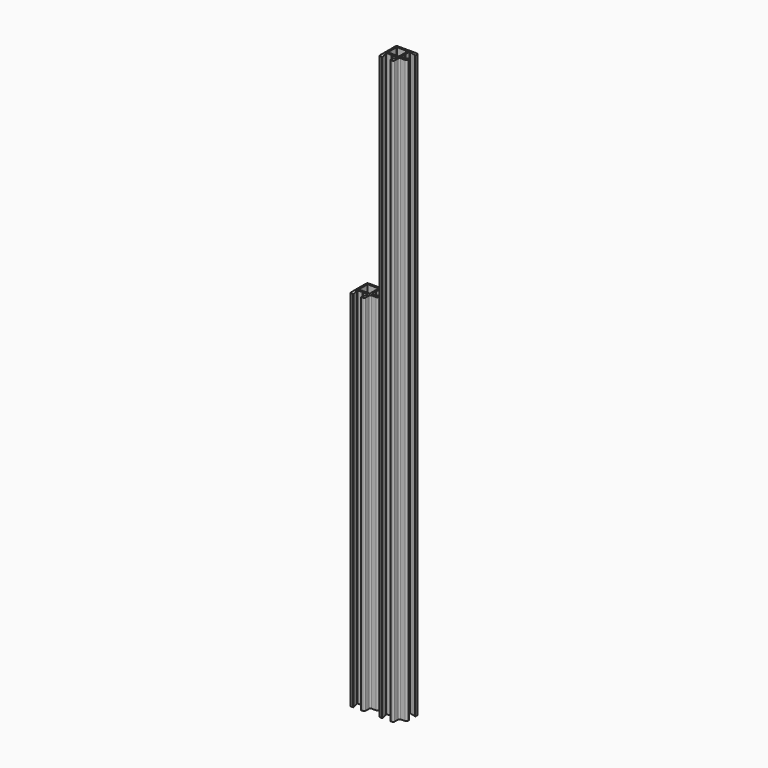
from build123d import *

# Parameters (mm, degrees)
F1_DEPTH = 1000
F2_DEPTH = 1600


# Not quite as in the source:
# - ends of sketch curves that miss each other by under 0.0002 mm in the source are joined


with BuildPart() as f1:
    # F0 (on Top) → F1 (new body)
    with BuildSketch(Plane.XY):
        with BuildLine():
            ThreePointArc((30, -1.879032), (29.5109517857, -0.8873403242), (28.4264761923, -0.6716247175))
            Line((28.4264761923, -0.6716247175), (11.258819, -5.271684))
            ThreePointArc((11.258819, -5.271684), (10.3912385359, -5.0991113133), (10, -4.305758))
            Line((10, -4.305758), (10, 9))
            ThreePointArc((10, 9), (9.9829629324, 9.1294094506), (9.9330127764, 9.2499998709))
            Line((9.9330127764, 9.2499998709), (9.644338, 9.75))
            ThreePointArc((9.644338, 9.75), (9.57735, 10), (9.6443374736, 10.2500003039))
            Line((9.6443374736, 10.2500003039), (9.933013, 10.75))
            ThreePointArc((9.933013, 10.75), (9.9829629324, 10.8705905494), (10, 11))
            Line((10, 11), (10, 24.305758))
            ThreePointArc((10, 24.305758), (10.3912385359, 25.0991113133), (11.2588189596, 25.2716838492))
            Line((11.2588189596, 25.2716838492), (28.426476, 20.671624))
            ThreePointArc((28.426476, 20.671624), (29.5109517857, 20.8873403242), (30, 21.879032))
            Line((30, 21.879032), (30, 26))
            ThreePointArc((30, 26), (28.8284271247, 28.8284271247), (26, 30))
            Line((26, 30), (-26, 30))
            ThreePointArc((-26, 30), (-28.8284271247, 28.8284271247), (-30, 26))
            Line((-30, 26), (-30, -26))
            ThreePointArc((-30, -26), (-28.8284271247, -28.8284271247), (-26, -30))
            Line((-26, -30), (-21.879032, -30))
            ThreePointArc((-21.879032, -30), (-20.8873403242, -29.5109517857), (-20.6716247175, -28.4264761923))
            Line((-20.6716247175, -28.4264761923), (-25.271684, -11.258819))
            ThreePointArc((-25.271684, -11.258819), (-25.0991113133, -10.3912385359), (-24.305758, -10))
            Line((-24.305758, -10), (-11, -10))
            ThreePointArc((-11, -10), (-10.8705905494, -9.9829629324), (-10.7500001291, -9.9330127764))
            Line((-10.7500001291, -9.9330127764), (-10.25, -9.644338))
            ThreePointArc((-10.25, -9.644338), (-10, -9.57735), (-9.7499996961, -9.6443374736))
            Line((-9.7499996961, -9.6443374736), (-9.25, -9.933013))
            ThreePointArc((-9.25, -9.933013), (-9.1294094506, -9.9829629324), (-9, -10))
            Line((-9, -10), (4.305758, -10))
            ThreePointArc((4.305758, -10), (5.0991113133, -10.3912385359), (5.2716838492, -11.2588189596))
            Line((5.2716838492, -11.2588189596), (0.671624, -28.426476))
            ThreePointArc((0.671624, -28.426476), (0.8873403242, -29.5109517857), (1.879032, -30))
            Line((1.879032, -30), (6, -30))
            ThreePointArc((6, -30), (8.8284271247, -28.8284271247), (10, -26))
            Line((10, -26), (10, -14))
            ThreePointArc((10, -14), (11.1715728753, -11.1715728753), (14, -10))
            Line((14, -10), (26, -10))
            ThreePointArc((26, -10), (28.8284271247, -8.8284271247), (30, -6))
            Line((30, -6), (30, -1.879032))
        make_face()
        with BuildLine():
            Line((5.25, 24.75), (5.25, -4.75))
            ThreePointArc((5.25, -4.75), (5.1035533906, -5.1035533906), (4.75, -5.25))
            Line((4.75, -5.25), (-24.75, -5.25))
            ThreePointArc((-24.75, -5.25), (-25.1035533906, -5.1035533906), (-25.25, -4.75))
            Line((-25.25, -4.75), (-25.25, 24.75))
            ThreePointArc((-25.25, 24.75), (-25.1035533906, 25.1035533906), (-24.75, 25.25))
            Line((-24.75, 25.25), (4.75, 25.25))
            ThreePointArc((4.75, 25.25), (5.1035533906, 25.1035533906), (5.25, 24.75))
        make_face(mode=Mode.SUBTRACT)
    extrude(amount=F1_DEPTH)


with BuildPart() as f2:
    # F0 (on Top) → F2 (new body)
    with BuildSketch(Plane.XY):
        with BuildLine():
            ThreePointArc((110, -1.879032), (109.5109517857, -0.8873403242), (108.4264761923, -0.6716247175))
            Line((108.4264761923, -0.6716247175), (91.258819, -5.271684))
            ThreePointArc((91.258819, -5.271684), (90.3912385359, -5.0991113133), (90, -4.305758))
            Line((90, -4.305758), (90, 9))
            ThreePointArc((90, 9), (89.9829629324, 9.1294094506), (89.9330127764, 9.2499998709))
            Line((89.9330127764, 9.2499998709), (89.644338, 9.75))
            ThreePointArc((89.644338, 9.75), (89.57735, 10), (89.6443374736, 10.2500003039))
            Line((89.6443374736, 10.2500003039), (89.933013, 10.75))
            ThreePointArc((89.933013, 10.75), (89.9829629324, 10.8705905494), (90, 11))
            Line((90, 11), (90, 24.305758))
            ThreePointArc((90, 24.305758), (90.3912385359, 25.0991113133), (91.2588189596, 25.2716838492))
            Line((91.2588189596, 25.2716838492), (108.426476, 20.671624))
            ThreePointArc((108.426476, 20.671624), (109.5109517857, 20.8873403242), (110, 21.879032))
            Line((110, 21.879032), (110, 26))
            ThreePointArc((110, 26), (108.8284271247, 28.8284271247), (106, 30))
            Line((106, 30), (54, 30))
            ThreePointArc((54, 30), (51.1715728753, 28.8284271247), (50, 26))
            Line((50, 26), (50, -26))
            ThreePointArc((50, -26), (51.1715728753, -28.8284271247), (54, -30))
            Line((54, -30), (58.120968, -30))
            ThreePointArc((58.120968, -30), (59.1126596758, -29.5109517857), (59.3283752825, -28.4264761923))
            Line((59.3283752825, -28.4264761923), (54.728316, -11.258819))
            ThreePointArc((54.728316, -11.258819), (54.9008886867, -10.3912385359), (55.694242, -10))
            Line((55.694242, -10), (69, -10))
            ThreePointArc((69, -10), (69.1294094506, -9.9829629324), (69.2499998709, -9.9330127764))
            Line((69.2499998709, -9.9330127764), (69.75, -9.644338))
            ThreePointArc((69.75, -9.644338), (70, -9.57735), (70.2500003039, -9.6443374736))
            Line((70.2500003039, -9.6443374736), (70.75, -9.933013))
            ThreePointArc((70.75, -9.933013), (70.8705905494, -9.9829629324), (71, -10))
            Line((71, -10), (84.305758, -10))
            ThreePointArc((84.305758, -10), (85.0991113133, -10.3912385359), (85.2716838492, -11.2588189596))
            Line((85.2716838492, -11.2588189596), (80.671624, -28.426476))
            ThreePointArc((80.671624, -28.426476), (80.8873403242, -29.5109517857), (81.879032, -30))
            Line((81.879032, -30), (86, -30))
            ThreePointArc((86, -30), (88.8284271247, -28.8284271247), (90, -26))
            Line((90, -26), (90, -14))
            ThreePointArc((90, -14), (91.1715728753, -11.1715728753), (94, -10))
            Line((94, -10), (106, -10))
            ThreePointArc((106, -10), (108.8284271247, -8.8284271247), (110, -6))
            Line((110, -6), (110, -1.879032))
        make_face()
        with BuildLine():
            Line((84.75, -5.25), (55.25, -5.25))
            ThreePointArc((55.25, -5.25), (54.8964466094, -5.1035533906), (54.75, -4.75))
            Line((54.75, -4.75), (54.75, 24.75))
            ThreePointArc((54.75, 24.75), (54.8964466094, 25.1035533906), (55.25, 25.25))
            Line((55.25, 25.25), (84.75, 25.25))
            ThreePointArc((84.75, 25.25), (85.1035533906, 25.1035533906), (85.25, 24.75))
            Line((85.25, 24.75), (85.25, -4.75))
            ThreePointArc((85.25, -4.75), (85.1035533906, -5.1035533906), (84.75, -5.25))
        make_face(mode=Mode.SUBTRACT)
    extrude(amount=F2_DEPTH)


solid = Compound([f1.part, f2.part])
